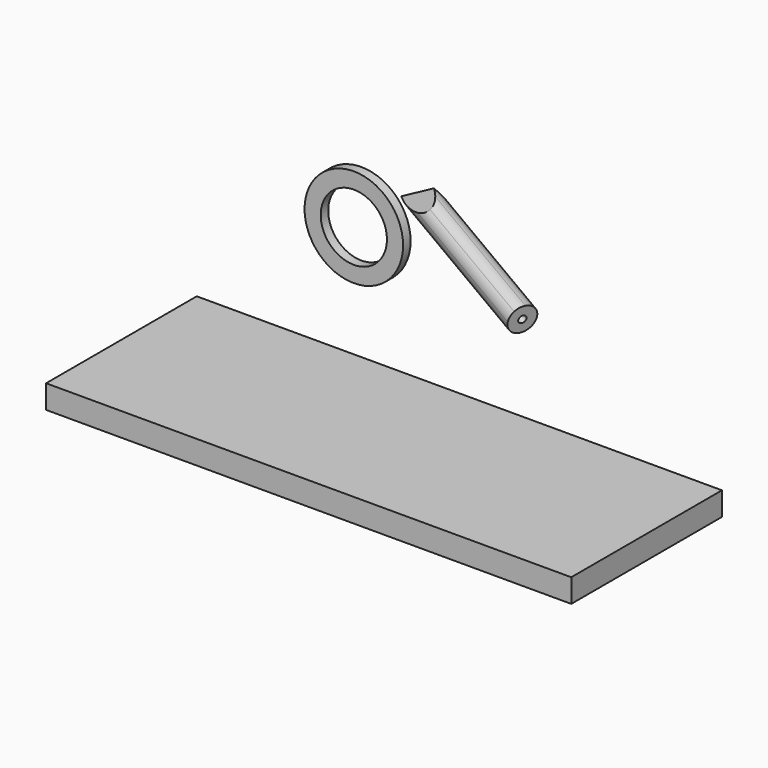
from build123d import *

# Parameters (mm, degrees)
F2_R      = 52.4468032927
F2_R_2    = 35.2687757181
F3_DEPTH  = 10
F9_W      = 20
F9_H      = 20
F9_R      = 4
F10_DEPTH = 2000
F11_DEPTH = 25
F13_W     = 559.1834336519
F13_H     = 200.5045488477
F14_DEPTH = 25
F16_W     = 3887.4027729034
F16_H     = 3285.4166030884
F18_DEPTH = 678.6163205323
F19_ANGLE = -225
F21_W     = 3887.4027729034
F21_H     = 3285.4166030884
F22_DEPTH = 38.8173766265


with BuildPart() as f3:
    # F2 (on offset) → F3 (new body)
    with BuildSketch(Plane.XZ.offset(-50)):
        Circle(F2_R)
        Circle(F2_R_2, mode=Mode.SUBTRACT)
    extrude(amount=F3_DEPTH)


with BuildPart() as f10:
    # F9 (on face) → F10 (new body)
    with BuildSketch(Plane(origin=(196.8001302702, -79.4746385064, -45.8847039354), x_dir=(0.3564382351, 0.9306155778, -0.0831049393), z_dir=(0.906307787, -0.3659981508, -0.2113091309))):
        with Locations((56.8793033835, 68.8264967326)):
            Rectangle(F9_W, F9_H)
        with Locations((56.8793033835, 68.8264967326)):
            Circle(F9_R, mode=Mode.SUBTRACT)
        with Locations((56.8793033835, 68.8264967326)):
            Circle(F9_R)
        with BuildLine():
            Line((46.8793033835, 58.8264967326), (46.8793033835, 78.8264967326))
            ThreePointArc((46.8793033835, 78.8264967326), (42.7371677598, 68.8264967326), (46.8793033835, 58.8264967326))
        make_face()
        with BuildLine():
            Line((46.8793033835, 78.8264967326), (66.8793033835, 78.8264967326))
            ThreePointArc((66.8793033835, 78.8264967326), (56.8793033835, 82.9686323564), (46.8793033835, 78.8264967326))
        make_face()
        with BuildLine():
            ThreePointArc((71.0214390072, 68.8264967326), (69.9449330323, 74.2384577341), (66.8793033835, 78.8264967326))
            Line((66.8793033835, 78.8264967326), (66.8793033835, 58.8264967326))
            ThreePointArc((66.8793033835, 58.8264967326), (69.9449330323, 63.4145357312), (71.0214390072, 68.8264967326))
        make_face()
        with BuildLine():
            ThreePointArc((46.8793033835, 58.8264967326), (56.8793033835, 54.6843611089), (66.8793033835, 58.8264967326))
            Line((66.8793033835, 58.8264967326), (46.8793033835, 58.8264967326))
        make_face()
    extrude(amount=-F10_DEPTH)

    # F9 (on face) → F11 (cut)
    with BuildSketch(Plane(origin=(196.8001302702, -79.4746385064, -45.8847039354), x_dir=(0.3564382351, 0.9306155778, -0.0831049393), z_dir=(0.906307787, -0.3659981508, -0.2113091309))):
        with Locations((56.8793033835, 68.8264967326)):
            Circle(F9_R)
    extrude(amount=-F11_DEPTH, mode=Mode.SUBTRACT)


with BuildPart() as f14:
    # F13 (on offset) → F14 (new body)
    with BuildSketch(Plane.XY.offset(-145)):
        with Locations((81.2806412578, -21.4358977973)):
            Rectangle(F13_W, F13_H)
    extrude(amount=-F14_DEPTH)


with BuildPart() as f10_1:
    # F17: moved
    add(f10.part)

    # F16 (on offset) → F18 (cut, through all)
    with BuildSketch(Plane.XZ.offset(-40)):
        with Locations((-28.5538434982, 86.0296487808)):
            Rectangle(F16_W, F16_H)
    extrude(amount=-F18_DEPTH, mode=Mode.SUBTRACT)


with BuildPart() as f10_2:
    # F19: moved
    add(f10_1.part.rotate(Axis((232.7020962549, -26.5418727237, 16.4170853719), (0.906307787, -0.3659981508, -0.2113091309)), F19_ANGLE))

    # F21 (on offset) → F22 (cut, through all)
    with BuildSketch(Plane.XZ.offset(-40)):
        with Locations((-28.5538434982, 86.0296487808)):
            Rectangle(F21_W, F21_H)
    extrude(amount=-F22_DEPTH, mode=Mode.SUBTRACT)


solid = Compound([f3.part, f14.part, f10_2.part])
